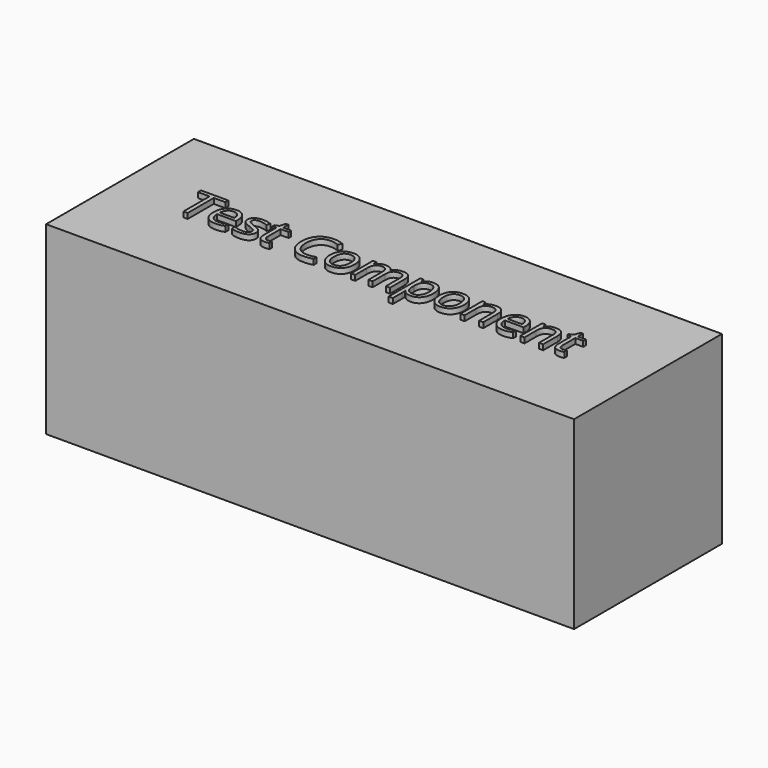
from build123d import *

# Parameters (mm, degrees)
F0_W         = 200
F0_H         = 70
F1_DEPTH     = 70
F3_TEXT_SIZE = 19.3007499146
F4_DEPTH     = 2


# Not quite as in the source:
# - Text() gives the source's letters only with a copy of the font that has no kerning and outlines rounded to 1/6400 em; it was checked with that copy


with BuildPart() as f1:
    # F0 (on Top) → F1 (new body)
    with BuildSketch(Plane.XY):
        Rectangle(F0_W, F0_H)
    extrude(amount=F1_DEPTH)

    # F3 (on offset) → F4 (join)
    with BuildSketch(Plane.XY.offset(70)):
        with Locations((-75.5060447348, -6.2394582827)):
            Text('Test Component', F3_TEXT_SIZE, font='Open Sans', text_align=(TextAlign.LEFT, TextAlign.BOTTOM))
    extrude(amount=F4_DEPTH)


solid = f1.part
